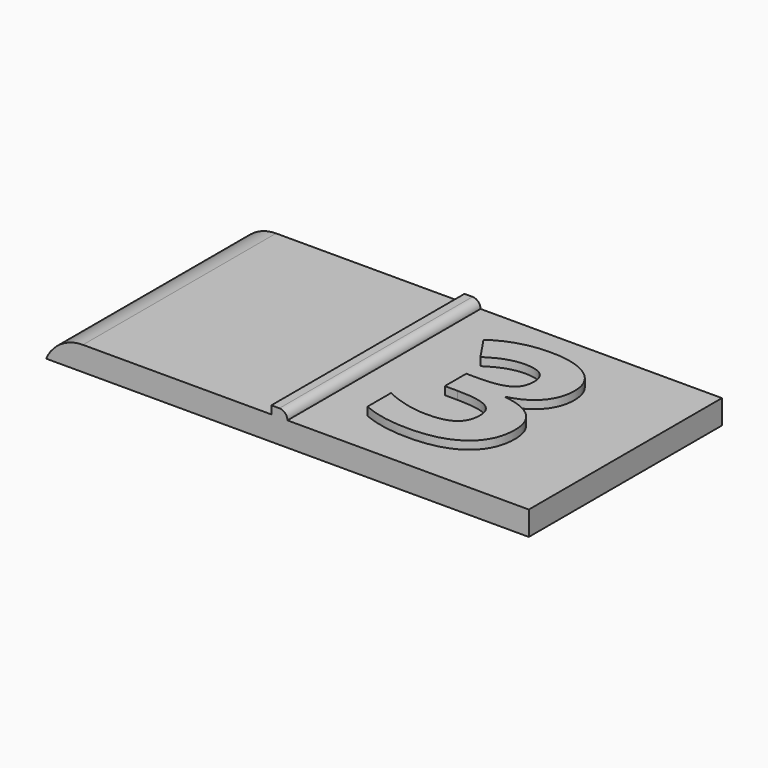
from build123d import *

# Parameters (mm, degrees)
F0_W         = 60
F0_H         = 30
F1_DEPTH     = 3
F2_W         = 2
F2_H         = 30
F3_DEPTH     = 1
F4_R         = 0.99999
F5_TEXT_SIZE = 28.8201948731
F6_DEPTH     = 1
F7_T1_DEPTH  = 52.9128784748


# Not quite as in the source:
# - a fillet or chamfer that OpenCascade refuses, or shapes differently, is made with other operations: its cross-section is extruded or revolved along the edge and cut away or added
# - a fillet or chamfer is up to 0.001 mm smaller than in the source, because OpenCascade refuses the exact size
# - Text() gives the source's letters only with a copy of the font that has no kerning and outlines rounded to 1/6400 em; it was checked with that copy


with BuildPart() as f1:
    # F0 (on Top) → F1 (new body)
    with BuildSketch(Plane.XY):
        with Locations((30, 15)):
            Rectangle(F0_W, F0_H)
    extrude(amount=F1_DEPTH)

    # F2 (on face) → F3 (join)
    with BuildSketch(Plane.XY.offset(3)):
        with Locations((29, 15)):
            Rectangle(F2_W, F2_H)
    extrude(amount=F3_DEPTH)

    # F4 (radius 1 in the source; OpenCascade refuses exactly that, so slightly less here)
    f4_edges = [f1.edges().sort_by_distance(p)[0] for p in [
        (30, 15, 4),
    ]]
    fillet(f4_edges, radius=F4_R)

    # F5 (on face) → F6 (join)
    with BuildSketch(Plane.XY.offset(3)):
        with Locations((34.3574509025, 4.7624194995)):
            Text('3', F5_TEXT_SIZE, font='Open Sans', font_style=FontStyle.BOLD, text_align=(TextAlign.LEFT, TextAlign.BOTTOM))
    extrude(amount=F6_DEPTH)

    # F7: fillet of radius 5 on 1 edges, made by hand

    # F7_s2 → F7_t1 (cut)
    with BuildSketch(Plane.XZ.offset(-41.4564392374)):
        with BuildLine():
            ThreePointArc((4.582575695, 3), (1.8439629074, 2.1833001327), (0, 0))
            Line((0, 0), (0, 3))
            Line((0, 3), (4.582575695, 3))
        make_face()
    extrude(amount=F7_T1_DEPTH, mode=Mode.SUBTRACT)


solid = f1.part
